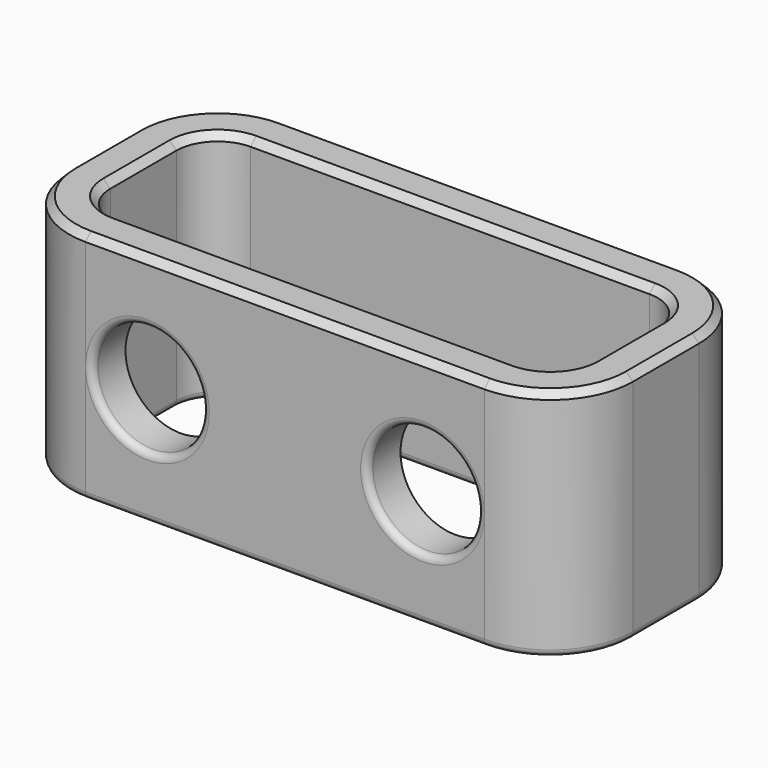
from build123d import *

# Parameters (mm, degrees)
F1_DEPTH = 17
F2_T     = -3
F3_R     = 4
F4_DEPTH = 5
F5_R     = 0.49999
F6_SIZE  = 0.5


# Not quite as in the source:
# - a fillet or chamfer is up to 0.001 mm smaller than in the source, because OpenCascade refuses the exact size


with BuildPart() as f1:
    # F0 (on Top) → F1 (new body)
    with BuildSketch(Plane.XY):
        with BuildLine():
            ThreePointArc((-20.5, -3), (-18.7426406871, -7.2426406871), (-14.5, -9))
            Line((-14.5, -9), (14.5, -9))
            ThreePointArc((14.5, -9), (18.7426406871, -7.2426406871), (20.5, -3))
            Line((20.5, -3), (20.5, 3))
            ThreePointArc((20.5, 3), (18.7426406871, 7.2426406871), (14.5, 9))
            Line((14.5, 9), (-14.5, 9))
            ThreePointArc((-14.5, 9), (-18.7426406871, 7.2426406871), (-20.5, 3))
            Line((-20.5, 3), (-20.5, -3))
        make_face()
    extrude(amount=F1_DEPTH)

    # F2
    f2_openings = [f1.faces().sort_by_distance(p)[0] for p in [
        (0, 0, 17),
        (0, 0, 0),
    ]]
    offset(amount=F2_T, openings=f2_openings)

    # F3 (on face) → F4 (cut)
    with BuildSketch(Plane.XZ.offset(9)):
        with Locations((-10, 8.5)):
            Circle(F3_R)
        with Locations((10, 8.5)):
            Circle(F3_R)
    extrude(amount=-F4_DEPTH, mode=Mode.SUBTRACT)

    # F5 (radius 0.5 in the source; OpenCascade refuses exactly that, so slightly less here)
    f5_edges = [f1.edges().sort_by_distance(p)[0] for p in [
        (0, 9, 0),
        (0, -6, 0),
        (6, -9, 8.5),
        (-14, -9, 8.5),
    ]]
    fillet(f5_edges, radius=F5_R)

    # F6
    f6_edges = [f1.edges().sort_by_distance(p)[0] for p in [
        (0, -9, 17),
        (0, -6, 17),
    ]]
    chamfer(f6_edges, length=F6_SIZE)


solid = f1.part
